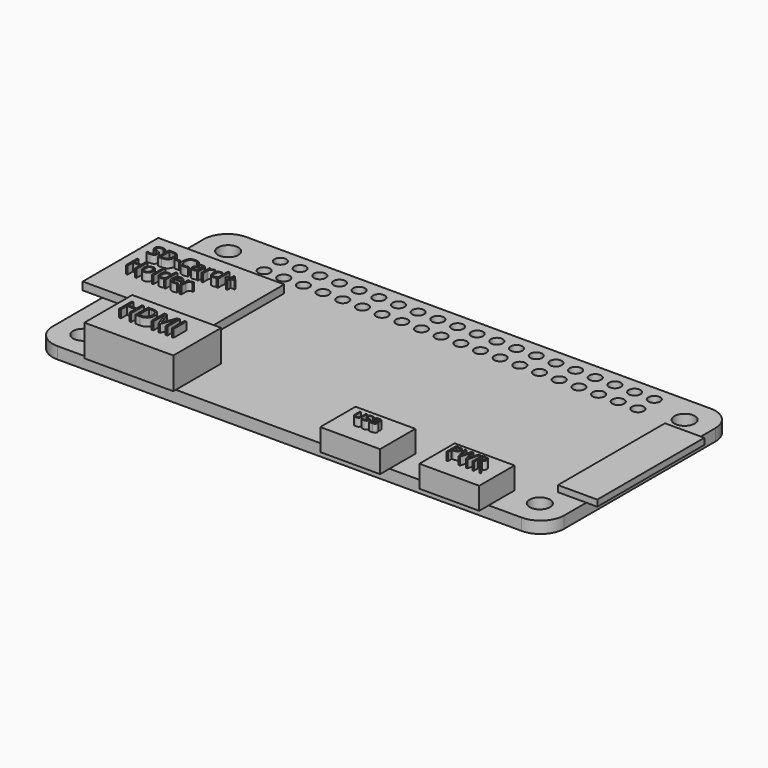
from build123d import *

# Parameters (mm, degrees)
F0_W            = 65
F0_H            = 30
F1_DEPTH        = 1.5
F2_R            = 1.3
F3_DEPTH        = 25
F4_R            = 3
F5_W            = 11.3
F5_H            = 7.6
F6_DEPTH        = 4
F7_W            = 7.6
F7_H            = 5.6
F8_DEPTH        = 2.8
F9_TEXT_SIZE    = 2.8205065367
F10_DEPTH       = 1
F11_TEXT_SIZE   = 1.6475471461
F11_TEXT_SIZE_2 = 2.1678266219
F12_DEPTH       = 1
F13_W           = 5
F13_H           = 17
F14_DEPTH       = 0.8
F15_W           = 16
F15_H           = 12
F16_DEPTH       = 1
F17_R           = 0.75
F18_DEPTH       = 25
F19_TEXT_SIZE   = 2.4791664651
F20_DEPTH       = 1


# Not quite as in the source:
# - Text() gives the source's letters only with a copy of the font that has no kerning and outlines rounded to 1/6400 em; it was checked with that copy


with BuildPart() as f1:
    # F0 (on Top) → F1 (new body)
    with BuildSketch(Plane.XY):
        Rectangle(F0_W, F0_H)
    extrude(amount=F1_DEPTH)

    # F2 (on face) → F3 (cut)
    with BuildSketch(Plane.XY.offset(1.5)):
        with Locations((-29, 11.5)):
            Circle(F2_R)
        with Locations((29, 11.5)):
            Circle(F2_R)
        with Locations((29, -11.5)):
            Circle(F2_R)
        with Locations((-29, -11.5)):
            Circle(F2_R)
    extrude(amount=-F3_DEPTH, mode=Mode.SUBTRACT)

    # F4
    f4_edges = [f1.edges().sort_by_distance(p)[0] for p in [
        (-32.5, 15, 0.75),
        (-32.5, -15, 0.75),
        (32.5, 15, 0.75),
        (32.5, -15, 0.75),
    ]]
    fillet(f4_edges, radius=F4_R)

    # F5 (on face) → F6 (join)
    with BuildSketch(Plane.XY.offset(1.5)):
        with Locations((-20.1, -11.6)):
            Rectangle(F5_W, F5_H)
    extrude(amount=F6_DEPTH)

    # F7 (on face) → F8 (join)
    with BuildSketch(Plane.XY.offset(1.5)):
        with Locations((8.9, -13.7)):
            Rectangle(F7_W, F7_H)
        with Locations((21.5, -13.7)):
            Rectangle(F7_W, F7_H)
    extrude(amount=F8_DEPTH)

    # F9 (on face) → F10 (join)
    with BuildSketch(Plane.XY.offset(5.5)):
        with Locations((-23.9947326481, -12.4179068953)):
            Text('HDMI', F9_TEXT_SIZE, font='Open Sans', text_align=(TextAlign.LEFT, TextAlign.BOTTOM))
    extrude(amount=F10_DEPTH)

    # F11 (on face) → F12 (join)
    with BuildSketch(Plane.XY.offset(4.3)):
        with Locations((7.1518654004, -14.1370333731)):
            Text('USB', F11_TEXT_SIZE, font='Open Sans', text_align=(TextAlign.LEFT, TextAlign.BOTTOM))
        with Locations((19.1702879965, -14.3243325874)):
            Text('PWR', F11_TEXT_SIZE_2, font='Open Sans', text_align=(TextAlign.LEFT, TextAlign.BOTTOM))
    extrude(amount=F12_DEPTH)

    # F13 (on face) → F14 (join)
    with BuildSketch(Plane.XY.offset(1.5)):
        with Locations((31.4, 0)):
            Rectangle(F13_W, F13_H)
    extrude(amount=F14_DEPTH)

    # F15 (on face) → F16 (join)
    with BuildSketch(Plane.XY.offset(1.5)):
        with Locations((-27, 1.9)):
            Rectangle(F15_W, F15_H)
    extrude(amount=F16_DEPTH)

    # F17 (on face) → F18 (cut)
    with BuildSketch(Plane.XY.offset(1.5)):
        with Locations((-23.5957577825, 13.0481310189)):
            Circle(F17_R)
        with Locations((-23.5957577825, 10.4481310189)):
            Circle(F17_R)
        with Locations((-21.0957577825, 13.0481310189)):
            Circle(F17_R)
        with Locations((-21.0957577825, 10.4481310189)):
            Circle(F17_R)
        with Locations((-18.5957577825, 13.0481310189)):
            Circle(F17_R)
        with Locations((-18.5957577825, 10.4481310189)):
            Circle(F17_R)
        with Locations((-16.0957577825, 13.0481310189)):
            Circle(F17_R)
        with Locations((-16.0957577825, 10.4481310189)):
            Circle(F17_R)
        with Locations((-13.5957577825, 13.0481310189)):
            Circle(F17_R)
        with Locations((-13.5957577825, 10.4481310189)):
            Circle(F17_R)
        with Locations((-11.0957577825, 13.0481310189)):
            Circle(F17_R)
        with Locations((-11.0957577825, 10.4481310189)):
            Circle(F17_R)
        with Locations((-8.5957577825, 13.0481310189)):
            Circle(F17_R)
        with Locations((-8.5957577825, 10.4481310189)):
            Circle(F17_R)
        with Locations((-6.0957577825, 13.0481310189)):
            Circle(F17_R)
        with Locations((-6.0957577825, 10.4481310189)):
            Circle(F17_R)
        with Locations((-3.5957577825, 13.0481310189)):
            Circle(F17_R)
        with Locations((-3.5957577825, 10.4481310189)):
            Circle(F17_R)
        with Locations((-1.0957577825, 13.0481310189)):
            Circle(F17_R)
        with Locations((-1.0957577825, 10.4481310189)):
            Circle(F17_R)
        with Locations((1.4042422175, 13.0481310189)):
            Circle(F17_R)
        with Locations((1.4042422175, 10.4481310189)):
            Circle(F17_R)
        with Locations((3.9042422175, 13.0481310189)):
            Circle(F17_R)
        with Locations((3.9042422175, 10.4481310189)):
            Circle(F17_R)
        with Locations((6.4042422175, 13.0481310189)):
            Circle(F17_R)
        with Locations((6.4042422175, 10.4481310189)):
            Circle(F17_R)
        with Locations((8.9042422175, 13.0481310189)):
            Circle(F17_R)
        with Locations((8.9042422175, 10.4481310189)):
            Circle(F17_R)
        with Locations((11.4042422175, 13.0481310189)):
            Circle(F17_R)
        with Locations((11.4042422175, 10.4481310189)):
            Circle(F17_R)
        with Locations((13.9042422175, 13.0481310189)):
            Circle(F17_R)
        with Locations((13.9042422175, 10.4481310189)):
            Circle(F17_R)
        with Locations((16.4042422175, 13.0481310189)):
            Circle(F17_R)
        with Locations((16.4042422175, 10.4481310189)):
            Circle(F17_R)
        with Locations((18.9042422175, 13.0481310189)):
            Circle(F17_R)
        with Locations((18.9042422175, 10.4481310189)):
            Circle(F17_R)
        with Locations((21.4042422175, 13.0481310189)):
            Circle(F17_R)
        with Locations((21.4042422175, 10.4481310189)):
            Circle(F17_R)
        with Locations((23.9042422175, 13.0481310189)):
            Circle(F17_R)
        with Locations((23.9042422175, 10.4481310189)):
            Circle(F17_R)
    extrude(amount=-F18_DEPTH, mode=Mode.SUBTRACT)

    # F19 (on face) → F20 (join)
    with BuildSketch(Plane.XY.offset(2.5)):
        with Locations((-32.8985024244, 3.1982299406)):
            Text('SD-Card+', F19_TEXT_SIZE, font='Open Sans', text_align=(TextAlign.LEFT, TextAlign.BOTTOM))
        with Locations((-32.8985024244, -0.1734364519)):
            Text('Holder', F19_TEXT_SIZE, font='Open Sans', text_align=(TextAlign.LEFT, TextAlign.BOTTOM))
    extrude(amount=F20_DEPTH)


solid = f1.part
